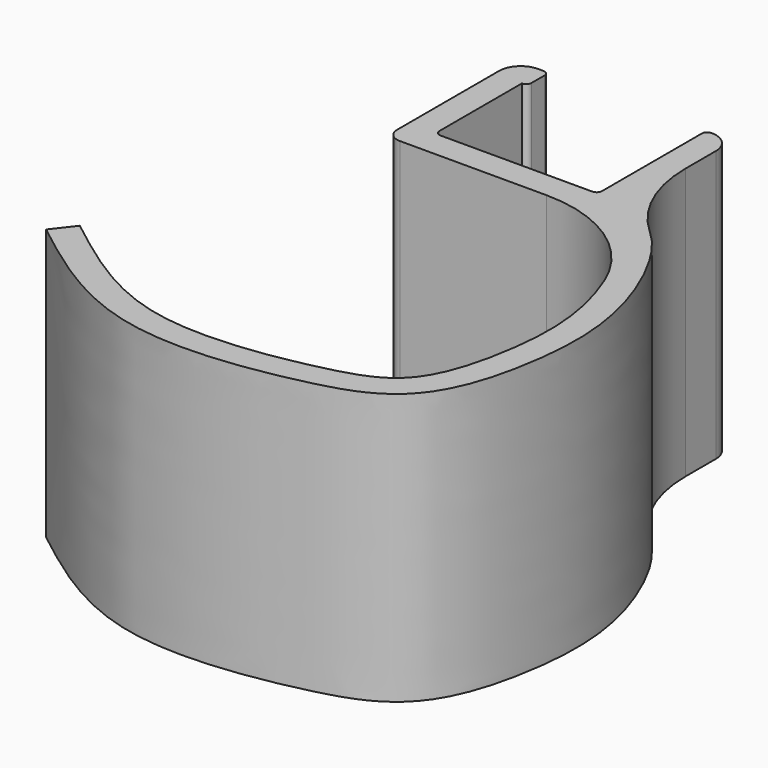
from build123d import *

# Parameters (mm, degrees)
F1_DEPTH = 10


# Not quite as in the source:
# - ends of sketch curves that miss each other by under 0.0002 mm in the source are joined
# - the dataset's text gives a spline's control points without its knots; the knots are read off the source's solid


with BuildPart() as f1:
    # F0 (on Top) → F1 (new body)
    with BuildSketch(Plane.XY):
        with BuildLine():
            Line((0, 4.8), (0, 0.8))
            Line((0, 0.8), (0, 0.2))
            ThreePointArc((0, 0.2), (-0.0585786438, 0.0585786438), (-0.2, 0))
            Line((-0.2, 0), (-0.8, 0))
            Line((-0.8, 0), (-5.8, 0))
            ThreePointArc((-5.8, 0), (-5.9414213562, 0.0585786438), (-6, 0.2))
            Line((-6, 0.2), (-6, 4))
            Line((-6, 4), (-6, 5))
            Line((-6, 5), (-6.2, 5))
            ThreePointArc((-6.2, 5), (-6.7656854249, 4.7656854249), (-7, 4.2))
            Line((-7, 4.2), (-7, -0.5))
            ThreePointArc((-7, -0.5), (-6.8535533906, -0.8535533906), (-6.5, -1))
            Line((-6.5, -1), (-2.3942277008, -1))
            Line((-2.3942277008, -1), (-1.0921858097, -1))
            ThreePointArc((-1.0921858097, -1), (1.6998635625, -1.8521740269), (3.540188152, -4.1182158786))
            add(Edge.make_bspline(
                [(3.540188152, -4.1182158786), (3.7375833678, -4.6041422119), (4.3405929184, -6.4657327179), (4.2192593573, -9.279113081), (3.2880898063, -12.6327405297), (0.5018426144, -13.5846985492), (-5.6234623598, -14.5743670196), (-8.8044643224, -12.1160958768), (-10.3983609006, -10.8843361959)],
                knots=[0.1895807753, 0.1895807753, 0.1895807753, 0.1895807753, 0.2440708291, 0.3883552133, 0.5187184375, 0.6404879891, 0.8198602294, 1, 1, 1, 1], degree=3))
            Line((-10.3983609006, -10.8843361959), (-11.0098433152, -11.6755942174))
            add(Edge.make_bspline(
                [(2.6623805568, -0.9237402788), (2.7011153859, -0.9584684447), (2.8325173821, -1.080318739), (3.0555325838, -1.3126427426), (3.3222089537, -1.6427920737), (3.6557618416, -2.1203124591), (4.0427641593, -2.7875133496), (4.4531495675, -3.6723207383), (4.7952161074, -4.6095497841), (5.13520119, -5.8951351698), (5.2543350057, -7.1378560018), (5.2116666311, -8.3267575258), (5.1142195068, -9.1939159274), (4.9710521005, -10.0412799545), (4.7709297659, -10.8986971922), (4.4898602262, -11.7308369468), (4.1618155742, -12.3856004901), (3.8159429164, -12.8708517403), (3.4060414781, -13.3139455927), (2.8156822247, -13.7394268291), (2.0466155042, -14.0804500091), (1.3687930436, -14.2824623359), (0.7976153994, -14.4242182099), (0.1918295557, -14.5630860717), (-0.6408356234, -14.7281188641), (-1.7244384375, -14.8851503279), (-2.8655768486, -14.9750498688), (-4.0368453172, -14.969108), (-5.016141336, -14.8587466142), (-5.7891223208, -14.6866401287), (-6.5315720354, -14.4626195491), (-7.4081890784, -14.0984319324), (-8.3854410649, -13.5625708051), (-9.6079497578, -12.7599743112), (-10.4568364151, -12.1029567026), (-11.0098433152, -11.6755942174)],
                knots=[0.0715908412, 0.0715908412, 0.0715908412, 0.0715908412, 0.078125, 0.09375, 0.109375, 0.125, 0.15625, 0.1875, 0.21875, 0.25, 0.3125, 0.34375, 0.375, 0.40625, 0.4375, 0.46875, 0.5, 0.515625, 0.53125, 0.5625, 0.59375, 0.625, 0.640625, 0.65625, 0.6875, 0.71875, 0.75, 0.78125, 0.8125, 0.828125, 0.84375, 0.875, 0.90625, 0.9375, 1, 1, 1, 1], degree=3))
            ThreePointArc((2.6623805568, -0.9237402788), (1.4344709504, 0.7605827051), (1, 2.7991960813))
            Line((1, 2.7991960813), (1, 4.2))
            ThreePointArc((1, 4.2), (0.7656854249, 4.7656854249), (0.2, 5))
            ThreePointArc((0.2, 5), (0.0585786438, 4.9414213562), (0, 4.8))
        make_face()
        with BuildLine():
            Line((-6, 5), (-6, 4))
            ThreePointArc((-6, 4), (-5.8585786438, 4.0585786438), (-5.8, 4.2))
            Line((-5.8, 4.2), (-5.8, 4.8))
            ThreePointArc((-5.8, 4.8), (-5.8585786438, 4.9414213562), (-6, 5))
        make_face()
    extrude(amount=-F1_DEPTH)


solid = f1.part
